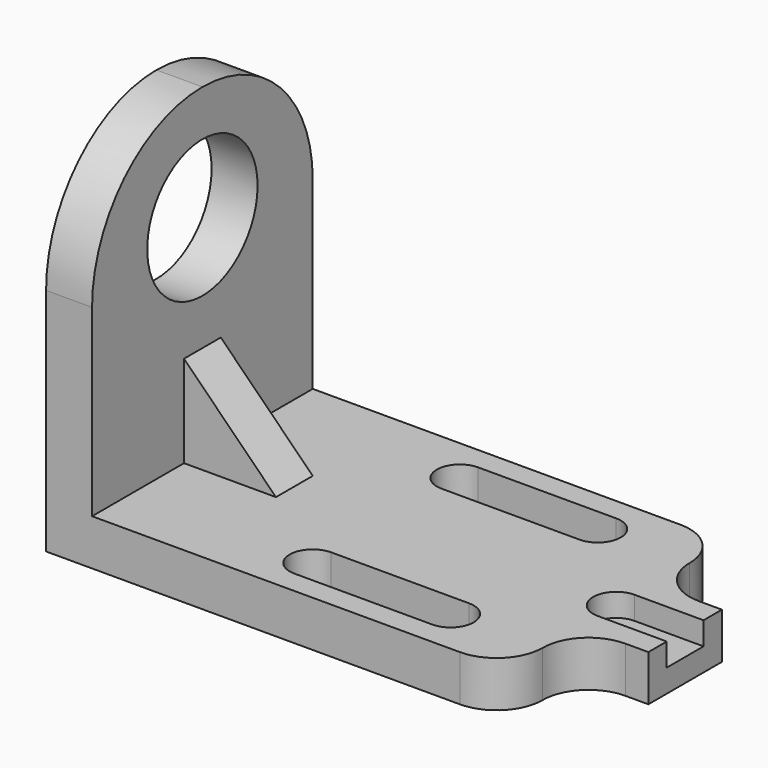
from build123d import *

# Parameters (mm, degrees)
F1_DEPTH  = 76.2
F2_DEPTH  = 12.7
F3_R      = 76.19999
F6_DEPTH  = 25.401
F7_DEPTH  = 25.401
F5_W      = 38.1
F5_H      = 12.7
F5_H_2    = 25.4
F8_DEPTH  = 25.4
F9_R      = 25.4
F10_R     = 25.39999
F11_DEPTH = 12.7


# Not quite as in the source:
# - a fillet or chamfer is up to 0.001 mm smaller than in the source, because OpenCascade refuses the exact size
# - a feature names something its author has since deleted; it is built from what else it names


with BuildPart() as f1:
    # F0 (on Front) → F1 (new body, symmetric)
    with BuildSketch(Plane.XZ):
        Polygon((0, 203.2), (0, 0), (254, 0), (254, 25.4), (76.2, 25.4), (25.4, 25.4), (25.4, 76.2), (25.4, 203.2), align=None)
    extrude(amount=F1_DEPTH, both=True)

    # F0 (on Front) → F2 (join, symmetric)
    with BuildSketch(Plane.XZ):
        Polygon((76.2, 25.4), (25.4, 76.2), (25.4, 25.4), align=None)
    extrude(amount=F2_DEPTH, both=True)

    # F3 (radius 76.2 in the source; OpenCascade refuses exactly that, so slightly less here)
    f3_edges = [f1.edges().sort_by_distance(p)[0] for p in [
        (12.7, -76.2, 203.2),
        (12.7, 76.2, 203.2),
    ]]
    fillet(f3_edges, radius=F3_R)

    # F5 (on face) → F6 (cut, through all)
    with BuildSketch(Plane.XY.offset(25.4)):
        with BuildLine():
            Line((203.2, 63.5), (127, 63.5))
            ThreePointArc((127, 63.5), (114.3, 50.8), (127, 38.1))
            Line((127, 38.1), (203.2, 38.1))
            ThreePointArc((203.2, 38.1), (215.9, 50.8), (203.2, 63.5))
        make_face()
        with BuildLine():
            Line((203.2, -38.1), (127, -38.1))
            ThreePointArc((127, -38.1), (114.3, -50.8), (127, -63.5))
            Line((127, -63.5), (203.2, -63.5))
            ThreePointArc((203.2, -63.5), (215.9, -50.8), (203.2, -38.1))
        make_face()
    extrude(amount=-F6_DEPTH, mode=Mode.SUBTRACT)

    # F4 (on face) → F7 (cut, through all)
    with BuildSketch(Plane.YZ.offset(25.4)):
        with BuildLine():
            Line((0, 101.6), (0, 177.8))
            ThreePointArc((0, 177.8), (-38.1, 139.7), (0, 101.6))
        make_face()
        with BuildLine():
            ThreePointArc((0, 101.6), (26.9407683632, 112.7592316368), (38.1, 139.7))
            ThreePointArc((38.1, 139.7), (26.9407683632, 166.6407683632), (0, 177.8))
            Line((0, 177.8), (0, 101.6))
        make_face()
    extrude(amount=-F7_DEPTH, mode=Mode.SUBTRACT)

    # F5 (on face) → F8 (join)
    with BuildSketch(Plane.XY.offset(25.4)):
        with Locations((273.05, 19.05)):
            Rectangle(F5_W, F5_H)
        with Locations((273.05, -19.05)):
            Rectangle(F5_W, F5_H)
        with Locations((273.05, 0)):
            Rectangle(F5_W, F5_H_2)
    extrude(amount=-F8_DEPTH)

    # F9
    f9_edges = [f1.edges().sort_by_distance(p)[0] for p in [
        (254, 76.2, 12.7),
        (254, -76.2, 12.7),
    ]]
    fillet(f9_edges, radius=F9_R)

    # F10 (radius 25.4 in the source; OpenCascade refuses exactly that, so slightly less here)
    f10_edges = [f1.edges().sort_by_distance(p)[0] for p in [
        (254, 25.4, 12.7),
        (254, -25.4, 12.7),
    ]]
    fillet(f10_edges, radius=F10_R)

    # F5 (on face) → F11 (cut)
    with BuildSketch(Plane.XY.offset(25.4)):
        with BuildLine():
            Line((254, -12.7), (254, 12.7))
            ThreePointArc((254, 12.7), (241.3, 0), (254, -12.7))
        make_face()
        with Locations((273.05, 0)):
            Rectangle(F5_W, F5_H_2)
    extrude(amount=-F11_DEPTH, mode=Mode.SUBTRACT)


solid = f1.part
